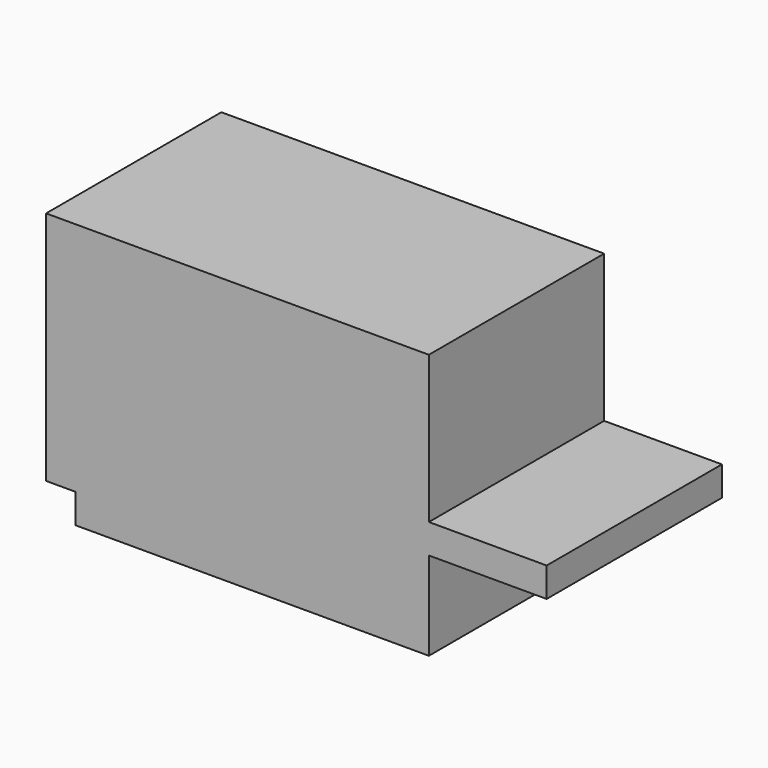
from build123d import *

# Parameters (mm, degrees)
F6_DEPTH = 47.244


# Not quite as in the source:
# - a feature of the source that left no trace in its solid (it failed there, or was rolled back) is left out


with BuildPart() as f6:
    # F0 (on Front) → F6 (new body)
    with BuildSketch(Plane.XZ):
        Polygon((52.8543624759, 44.45), (-29.6956375241, 44.45), (-29.6956375241, -6.35), (-23.3456375241, -6.35), (-23.3456375241, -12.7), (52.8543624759, -12.7), (52.8543624759, 6.35), (78.2543624759, 6.35), (78.2543624759, 12.7), (52.8543624759, 12.7), align=None)
    extrude(amount=-F6_DEPTH)


solid = f6.part
